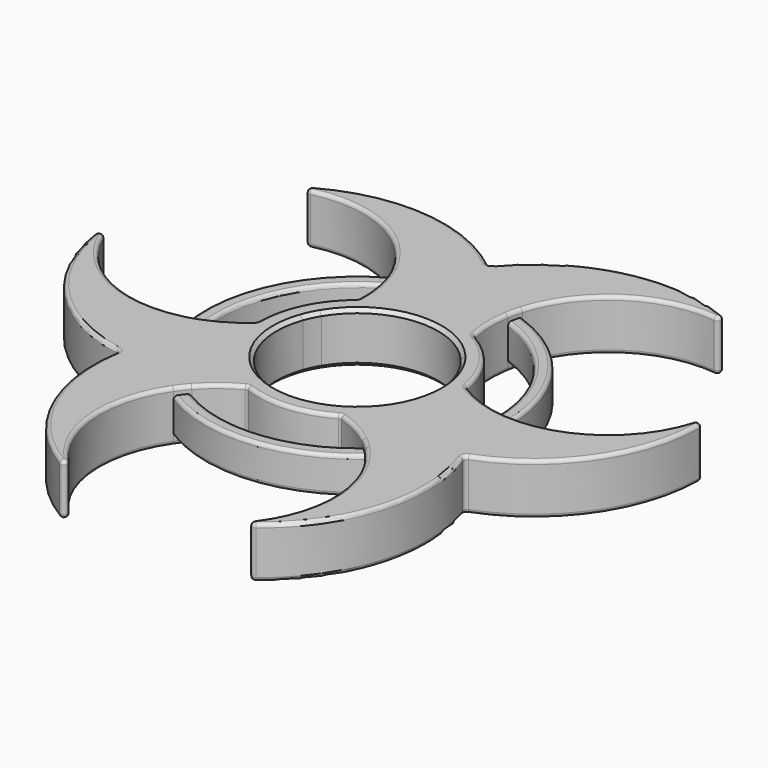
from build123d import *

# Parameters (mm, degrees)
F1_DEPTH  = 7
F2_DEPTH  = 5
F3_R      = 0.5
F4_SIZE   = 0.5
F6_R      = 0.5
F6_2_R    = 0.5
F6_3_R    = 0.5
F7_R      = 11.25
F7_R_2    = 5
F8_DEPTH  = 2
F7_R_3    = 3.8
F9_DEPTH  = 3
F7_R_4    = 1.5
F10_DEPTH = 6.25
F11_R     = 0.49999
F12_SIZE  = 0.5


# Not quite as in the source:
# - a fillet or chamfer is up to 0.001 mm smaller than in the source, because OpenCascade refuses the exact size


with BuildPart() as f1:
    # F0 (on Top) → F1 (new body)
    with BuildSketch(Plane.XY):
        with BuildLine():
            ThreePointArc((-9.735489, -16.316257), (-7.544062, -14.271114), (-5.009632, -12.670604))
            ThreePointArc((-5.009632, -12.670604), (1.12339, -13.578609), (7.023804, -11.67505))
            ThreePointArc((7.023804, -11.67505), (9.786803, -12.837291), (12.284534, -14.494489))
            ThreePointArc((12.284534, -14.494489), (13.047956, -15.15213), (13.768469, -15.856521))
            ThreePointArc((13.768469, -15.856521), (18.195807, -27.966303), (12.254047, -39.409365))
            ThreePointArc((12.254047, -39.409365), (23.254529, -27.159937), (23.261749, -10.696067))
            ThreePointArc((23.261749, -10.696067), (35.372481, -0.653239), (38.205602, 14.822602))
            ThreePointArc((38.205602, 14.822602), (32.875021, 3.467449), (20.992713, -0.553166))
            ThreePointArc((20.992713, -0.553166), (19.990963, -0.444529), (18.998038, -0.273052))
            ThreePointArc((18.998038, -0.273052), (16.131178, 0.602208), (13.477881, 1.996834))
            ThreePointArc((13.477881, 1.996834), (11.197725, 7.762189), (6.598988, 11.920318))
            ThreePointArc((6.598988, 11.920318), (6.224019, 14.894266), (6.410329, 17.885963))
            ThreePointArc((6.410329, 17.885963), (6.598152, 18.875927), (6.847915, 19.852105))
            ThreePointArc((6.847915, 19.852105), (15.121626, 29.741183), (28.002487, 30.316998))
            ThreePointArc((28.002487, 30.316998), (11.893931, 33.718981), (-2.367809, 25.493299))
            ThreePointArc((-2.367809, 25.493299), (-17.120519, 30.960086), (-31.939551, 25.675721))
            ThreePointArc((-31.939551, 25.675721), (-19.440409, 26.736879), (-10.017301, 18.456806))
            ThreePointArc((-10.017301, 18.456806), (-9.610508, 17.534947), (-9.262549, 16.58931))
            ThreePointArc((-9.262549, 16.58931), (-8.587116, 13.668906), (-8.468249, 10.673771))
            ThreePointArc((-8.468249, 10.673771), (-12.321115, 5.81642), (-13.622792, -0.245268))
            ThreePointArc((-13.622792, -0.245268), (-16.010822, -2.056975), (-18.694863, -3.391474))
            ThreePointArc((-18.694863, -3.391474), (-19.646108, -3.723796), (-20.616385, -3.995584))
            ThreePointArc((-20.616385, -3.995584), (-33.317433, -1.774879), (-40.256534, 9.092366))
            ThreePointArc((-40.256534, 9.092366), (-35.14846, -6.559044), (-20.89394, -14.797232))
            ThreePointArc((-20.89394, -14.797232), (-18.251962, -30.306847), (-6.266051, -40.498323))
            ThreePointArc((-6.266051, -40.498323), (-13.434612, -30.204328), (-10.975413, -17.90364))
            ThreePointArc((-10.975413, -17.90364), (-10.380455, -17.090417), (-9.735489, -16.316257))
        make_face()
        with BuildLine():
            ThreePointArc((9.727704, 5.397906), (10.770012, 2.787913), (11.125, 0))
            ThreePointArc((11.125, 0), (8.549203, -7.11876), (2.014573, -10.941075))
            ThreePointArc((2.014573, -10.941075), (0.917263, -11.087121), (-0.189128, -11.123392))
            ThreePointArc((-0.189128, -11.123392), (-9.143097, -6.337934), (-10.482535, 3.725866))
            ThreePointArc((-10.482535, 3.725866), (-10.06036, 4.749187), (-9.538576, 5.725486))
            ThreePointArc((-9.538576, 5.725486), (-0.917263, 11.087121), (8.467962, 7.215209))
            ThreePointArc((8.467962, 7.215209), (9.143097, 6.337934), (9.727704, 5.397906))
        make_face(mode=Mode.SUBTRACT)
    extrude(amount=F1_DEPTH)

    # F3
    f3_edges = [f1.edges().sort_by_distance(p)[0] for p in [
        (29.582903, 1.196863, 7),
        (-29.738401, -3.559293, 7),
        (-17.120519, 30.960086, 7),
        (23.254529, -27.159937, 0),
        (17.951639, -23.974564, 7),
        (-17.120519, 30.960086, 0),
        (35.372481, -0.653239, 0),
        (-18.251962, -30.306847, 7),
        (-2.367809, 25.493299, 3.5),
        (11.786762, 27.533858, 7),
        (-12.321115, 5.81642, 0),
        (-15.827966, 25.021114, 7),
        (1.12339, -13.578609, 7),
        (11.893931, 33.718981, 7),
        (11.786762, 27.533858, 0),
        (35.372481, -0.653239, 7),
        (11.197725, 7.762189, 7),
        (-13.754938, -26.217977, 0),
        (-29.738401, -3.559293, 0),
        (23.254529, -27.159937, 7),
        (-12.321115, 5.81642, 7),
        (-13.754938, -26.217977, 7),
        (29.582903, 1.196863, 0),
        (11.893931, 33.718981, 0),
        (11.197725, 7.762189, 0),
        (-35.14846, -6.559044, 7),
        (6.598988, 11.920318, 3.5),
        (38.205602, 14.822602, 3.5),
        (-20.89394, -14.797232, 3.5),
        (-35.14846, -6.559044, 0),
        (-8.468249, 10.673771, 3.5),
        (1.12339, -13.578609, 0),
        (-15.827966, 25.021114, 0),
        (7.023804, -11.67505, 3.5),
        (13.477881, 1.996834, 3.5),
        (-13.622792, -0.245268, 3.5),
        (-6.266051, -40.498323, 3.5),
        (12.254047, -39.409365, 3.5),
        (-31.939551, 25.675721, 3.5),
        (28.002487, 30.316998, 3.5),
        (17.951639, -23.974564, 0),
        (-18.251962, -30.306847, 0),
        (-5.009632, -12.670604, 3.5),
        (23.261749, -10.696067, 3.5),
        (-40.256534, 9.092366, 3.5),
    ]]
    fillet(f3_edges, radius=F3_R)

    # F4
    f4_edges = [f1.edges().sort_by_distance(p)[0] for p in [
        (-2.014573, 10.941075, 7),
        (-2.014573, 10.941075, 0),
    ]]
    chamfer(f4_edges, length=F4_SIZE)


with BuildPart() as f2:
    # F0 (on Top) → F2 (new body)
    with BuildSketch(Plane.XY):
        with BuildLine():
            ThreePointArc((12.284534, -14.494489), (1.566562, -18.935308), (-9.735489, -16.316257))
            ThreePointArc((-9.735489, -16.316257), (-10.380455, -17.090417), (-10.975413, -17.90364))
            ThreePointArc((-10.975413, -17.90364), (1.731463, -20.928498), (13.768469, -15.856521))
            ThreePointArc((13.768469, -15.856521), (13.047956, -15.15213), (12.284534, -14.494489))
        make_face()
    extrude(amount=-F2_DEPTH)


with BuildPart() as f2b:
    # F0 (on Top) → F2, piece 2 (new body)
    with BuildSketch(Plane.XY):
        with BuildLine():
            ThreePointArc((-10.017301, 18.456806), (-18.990343, 8.964758), (-20.616385, -3.995584))
            ThreePointArc((-20.616385, -3.995584), (-19.646108, -3.723796), (-18.694863, -3.391474))
            ThreePointArc((-18.694863, -3.391474), (-17.181739, 8.110971), (-9.262549, 16.58931))
            ThreePointArc((-9.262549, 16.58931), (-9.610508, 17.534947), (-10.017301, 18.456806))
        make_face()
    extrude(amount=-F2_DEPTH)


with BuildPart() as f2c:
    # F0 (on Top) → F2, piece 3 (new body)
    with BuildSketch(Plane.XY):
        with BuildLine():
            ThreePointArc((18.998038, -0.273052), (19.990963, -0.444529), (20.992713, -0.553166))
            ThreePointArc((20.992713, -0.553166), (17.258879, 11.96374), (6.847915, 19.852105))
            ThreePointArc((6.847915, 19.852105), (6.598152, 18.875927), (6.410329, 17.885963))
            ThreePointArc((6.410329, 17.885963), (15.615177, 10.824336), (18.998038, -0.273052))
        make_face()
    extrude(amount=-F2_DEPTH)


with BuildPart() as f2b_1:
    # F5: moved
    add(f2b.part.moved(Location((0, 0, 6))))

    # F6
    f6_edges = [f2b_1.edges().sort_by_distance(p)[0] for p in [
        (-18.990343, 8.964758, 6),
        (-17.181739, 8.110971, 1),
        (-17.181739, 8.110971, 6),
        (-18.990343, 8.964758, 1),
    ]]
    fillet(f6_edges, radius=F6_R)


with BuildPart() as f2c_1:
    # F5: moved
    add(f2c.part.moved(Location((0, 0, 6))))

    # F6#3
    f6_3_edges = [f2c_1.edges().sort_by_distance(p)[0] for p in [
        (17.258879, 11.96374, 6),
        (15.615177, 10.824336, 6),
        (17.258879, 11.96374, 1),
        (15.615177, 10.824336, 1),
    ]]
    fillet(f6_3_edges, radius=F6_3_R)


with BuildPart() as f2_1:
    # F5: moved
    add(f2.part.moved(Location((0, 0, 6))))

    # F6#2
    f6_2_edges = [f2_1.edges().sort_by_distance(p)[0] for p in [
        (1.731463, -20.928498, 1),
        (1.731463, -20.928498, 6),
        (1.566562, -18.935308, 6),
        (1.566562, -18.935308, 1),
    ]]
    fillet(f6_2_edges, radius=F6_2_R)


with BuildPart() as f8:
    # F7 (on Top) → F8 (new body)
    with BuildSketch(Plane.XY):
        with Locations((26.497496, 19.515725)):
            Circle(F7_R)
        with Locations((26.497496, 19.515725)):
            Circle(F7_R_2, mode=Mode.SUBTRACT)
    extrude(amount=F8_DEPTH)

    # F7 (on Top) → F9 (join)
    with BuildSketch(Plane.XY):
        with Locations((26.497496, 19.515725)):
            Circle(F7_R_2)
        with Locations((26.497496, 19.515725)):
            Circle(F7_R_3, mode=Mode.SUBTRACT)
    extrude(amount=F9_DEPTH)

    # F7 (on Top) → F10 (join)
    with BuildSketch(Plane.XY):
        with Locations((26.497496, 19.515725)):
            Circle(F7_R_3)
        with Locations((26.497496, 19.515725)):
            Circle(F7_R_4, mode=Mode.SUBTRACT)
    extrude(amount=F10_DEPTH)

    # F11 (radius 0.5 in the source; OpenCascade refuses exactly that, so slightly less here)
    f11_edges = [f8.edges().sort_by_distance(p)[0] for p in [
        (24.997496, 19.515725, 6.25),
        (15.247496, 19.515725, 2),
        (21.497496, 19.515725, 3),
        (21.497496, 19.515725, 2),
        (15.247496, 19.515725, 0),
        (24.997496, 19.515725, 0),
    ]]
    fillet(f11_edges, radius=F11_R)

    # F12
    f12_edges = [f8.edges().sort_by_distance(p)[0] for p in [
        (22.697496, 19.515725, 6.25),
    ]]
    chamfer(f12_edges, length=F12_SIZE)


solid = Compound([f1.part, f2b_1.part, f2c_1.part, f2_1.part])
